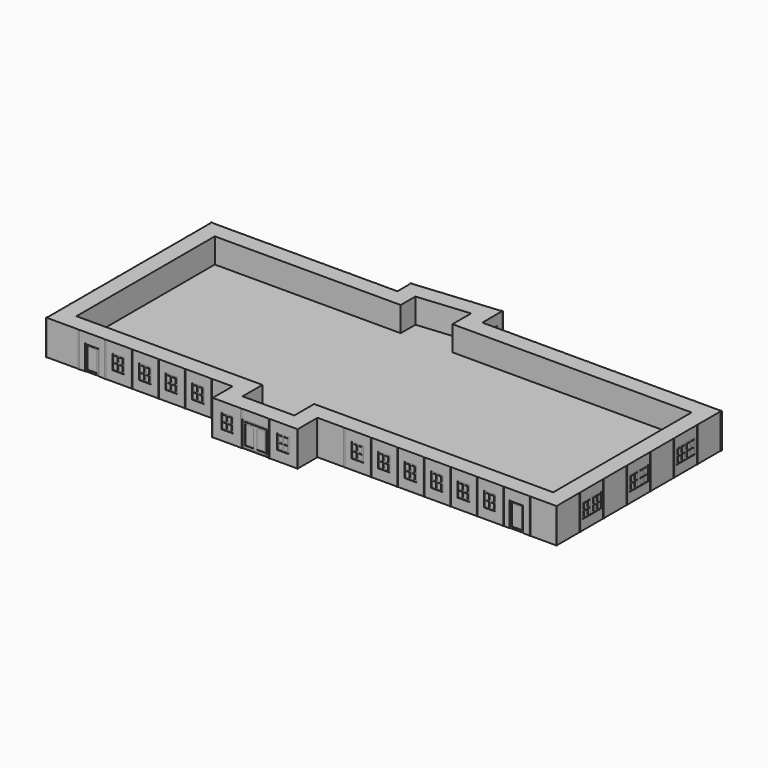
from build123d import *

# Parameters (mm, degrees)
F1_DEPTH  = 42
F3_DEPTH  = 30
F4_W      = 1.6
F4_H      = 42
F4_W_2    = 0.8
F6_W      = 1.6
F6_H      = 42
F8_W      = 1.6
F8_H      = 42
F8_W_2    = 0.8
F16_DEPTH = 0.4
F5_W      = 0.8
F5_H      = 42
F5_W_2    = 1.6
F10_W     = 1.6
F10_H     = 42
F12_W     = 0.8
F12_H     = 42
F12_W_2   = 1.6
F17_DEPTH = 0.4
F7_W      = 0.8
F7_H      = 42
F7_W_2    = 1.6
F9_W      = 1.6
F9_H      = 42
F14_W     = 0.8
F14_H     = 42
F14_W_2   = 1.6
F18_DEPTH = 0.4
F11_W     = 1.6
F11_H     = 42
F11_W_2   = 0.8
F13_W     = 1.6
F13_H     = 42
F15_W     = 1.6
F15_H     = 42
F15_W_2   = 0.8
F19_DEPTH = 0.4
F20_W     = 14.1428571429
F20_H     = 18
F20_W_2   = 4.1785714286
F20_H_2   = 6.1071428571
F21_W     = 14.1428571429
F21_H     = 18
F21_W_2   = 4.1785714286
F21_H_2   = 6.1071428571
F22_W     = 14.1428571429
F22_H     = 18
F22_W_2   = 4.1785714286
F22_H_2   = 6.1071428571
F23_DEPTH = 0.5
F24_W     = 17
F24_H     = 30
F24_W_2   = 15
F24_H_2   = 28
F24_W_3   = 12
F24_H_3   = 25
F25_DEPTH = 0.5
F26_W     = 17
F26_H     = 30
F26_W_2   = 15
F26_H_2   = 28
F26_W_3   = 12
F26_H_3   = 25
F27_DEPTH = 0.5
F28_W     = 31.4
F28_H     = 31
F28_W_2   = 27.4
F28_H_2   = 27
F28_W_3   = 10
F28_H_3   = 23
F29_DEPTH = 0.5
F32_W     = 14.1428571429
F32_H     = 18
F32_W_2   = 4.1785714286
F32_H_2   = 6.1071428571
F31_W     = 14.1428571429
F31_H     = 18
F31_W_2   = 4.1785714286
F31_H_2   = 6.1071428571
F30_W     = 14.1428571429
F30_H     = 18
F30_W_2   = 4.1785714286
F30_H_2   = 6.1071428571
F33_DEPTH = 0.5
F34_W     = 17
F34_H     = 30
F34_W_2   = 15
F34_H_2   = 28
F34_W_3   = 12
F34_H_3   = 25
F35_DEPTH = 0.5
F36_W     = 14.1428571429
F36_H     = 18
F36_W_2   = 4.1785714286
F36_H_2   = 6.1071428571
F37_W     = 30.4
F37_H     = 31
F37_W_2   = 26.4
F37_H_2   = 27
F37_W_3   = 10
F37_H_3   = 23
F38_DEPTH = 0.5
F39_W     = 4.1785714286
F39_H     = 6.1071428571
F39_W_2   = 14.1428571429
F39_H_2   = 18
F40_DEPTH = 0.5
F41_W     = 14.1428571429
F41_H     = 18
F41_W_2   = 4.1785714286
F41_H_2   = 6.1071428571
F42_DEPTH = 0.5
F43_W     = 14.1428571429
F43_H     = 18
F43_W_2   = 4.1785714286
F43_H_2   = 6.1071428571
F44_DEPTH = 0.5


# Not quite as in the source:
# - a feature names something its author has since deleted; it is built from what else it names


with BuildPart() as f1:
    # F0 (on Top) → F1 (new body)
    with BuildSketch(Plane.XY):
        Polygon((-327.3, 108.1424002851), (-327.3, -140.8575997149), (-102.6, -140.8575997149), (-102.6, -170.8575997149), (0, -170.8575997149), (0, -140.8575997149), (288.9, -140.8575997149), (288.9, 108.1424002851), (0, 108.1424002851), (0, 138.1424002851), (-102.6, 128.6424002851), (-102.6, 108.1424002851), align=None)
    extrude(amount=F1_DEPTH)

    # F2 (on face) → F3 (cut)
    with BuildSketch(Plane.XY.offset(42)):
        Polygon((-20, 88.1424002851), (-20, 116.2049975252), (-82.6, 110.4087012289), (-82.6, 88.1424002851), (-307.3, 88.1424002851), (-307.3, -120.8575997149), (-82.6, -120.8575997149), (-82.6, -150.8575997149), (-20, -150.8575997149), (-20, -120.8575997149), (268.9, -120.8575997149), (268.9, 88.1424002851), align=None)
    extrude(amount=-F3_DEPTH, mode=Mode.SUBTRACT)

    # F4 (on face) + F6 (on face) + F8 (on face) → F16 (join)
    with BuildSketch(Plane.XZ.offset(140.8575997149)):
        with Locations((-288.375, 21)):
            Rectangle(F4_W, F4_H)
        with Locations((-256.375, 21)):
            Rectangle(F4_W, F4_H)
        with Locations((-224.375, 21)):
            Rectangle(F4_W, F4_H)
        with Locations((-192.375, 21)):
            Rectangle(F4_W, F4_H)
        with Locations((-160.375, 21)):
            Rectangle(F4_W, F4_H)
        with Locations((-128.375, 21)):
            Rectangle(F4_W, F4_H)
        with Locations((-103, 21)):
            Rectangle(F4_W_2, F4_H)
        with Locations((-326.9, 21)):
            Rectangle(F4_W, F4_H)
    with BuildSketch(Plane.XZ.offset(170.8575997149)):
        with Locations((-102.2, 21)):
            Rectangle(F6_W, F6_H)
        with Locations((-0.4, 21)):
            Rectangle(F6_W, F6_H)
        with Locations((-34.8, 21)):
            Rectangle(F6_W, F6_H)
        with Locations((-67.8, 21)):
            Rectangle(F6_W, F6_H)
    with BuildSketch(Plane.XZ.offset(140.8575997149)):
        with Locations((288.5, 21)):
            Rectangle(F8_W, F8_H)
        with Locations((256.5, 21)):
            Rectangle(F8_W, F8_H)
        with Locations((224.5, 21)):
            Rectangle(F8_W, F8_H)
        with Locations((192.5, 21)):
            Rectangle(F8_W, F8_H)
        with Locations((160.5, 21)):
            Rectangle(F8_W, F8_H)
        with Locations((128.5, 21)):
            Rectangle(F8_W, F8_H)
        with Locations((96.5, 21)):
            Rectangle(F8_W, F8_H)
        with Locations((64.5, 21)):
            Rectangle(F8_W, F8_H)
        with Locations((32.5, 21)):
            Rectangle(F8_W, F8_H)
        with Locations((0.4, 21)):
            Rectangle(F8_W_2, F8_H)
    extrude(amount=F16_DEPTH)

    # F5 (on face) + F10 (on face) + F12 (on face) → F17 (join)
    with BuildSketch(Plane(origin=(-102.6, 0, 0), x_dir=(0, -1, 0), z_dir=(-1, 0, 0))):
        with Locations((141.2575997149, 21)):
            Rectangle(F5_W, F5_H)
        with Locations((170.4575997149, 21)):
            Rectangle(F5_W_2, F5_H)
    with BuildSketch(Plane(origin=(-327.3, 0, 0), x_dir=(0, -1, 0), z_dir=(-1, 0, 0))):
        with Locations((-108.0424002851, 21)):
            Rectangle(F10_W, F10_H)
        with Locations((-72.5424002851, 21)):
            Rectangle(F10_W, F10_H)
        with Locations((-37.0424002851, 21)):
            Rectangle(F10_W, F10_H)
        with Locations((-1.5424002851, 21)):
            Rectangle(F10_W, F10_H)
        with Locations((33.9575997149, 21)):
            Rectangle(F10_W, F10_H)
        with Locations((69.4575997149, 21)):
            Rectangle(F10_W, F10_H)
        with Locations((104.9575997149, 21)):
            Rectangle(F10_W, F10_H)
        with Locations((140.4575997149, 21)):
            Rectangle(F10_W, F10_H)
    with BuildSketch(Plane(origin=(-102.6, 0, 0), x_dir=(0, -1, 0), z_dir=(-1, 0, 0))):
        with Locations((-108.5424002851, 21)):
            Rectangle(F12_W, F12_H)
        with Locations((-128.2424002851, 21)):
            Rectangle(F12_W_2, F12_H)
    extrude(amount=F17_DEPTH)

    # F7 (on face) + F9 (on face) + F14 (on face) → F18 (join)
    with BuildSketch(Plane.YZ):
        with Locations((-141.2575997149, 21)):
            Rectangle(F7_W, F7_H)
        with Locations((-170.4575997149, 21)):
            Rectangle(F7_W_2, F7_H)
    with BuildSketch(Plane.YZ.offset(288.9)):
        with Locations((-140.4575997149, 21)):
            Rectangle(F9_W, F9_H)
        with Locations((-105.0004568577, 21)):
            Rectangle(F9_W, F9_H)
        with Locations((-69.5433140006, 21)):
            Rectangle(F9_W, F9_H)
        with Locations((-34.0861711434, 21)):
            Rectangle(F9_W, F9_H)
        with Locations((1.3709717137, 21)):
            Rectangle(F9_W, F9_H)
        with Locations((36.8281145709, 21)):
            Rectangle(F9_W, F9_H)
        with Locations((72.285257428, 21)):
            Rectangle(F9_W, F9_H)
        with Locations((107.7424002851, 21)):
            Rectangle(F9_W, F9_H)
    with BuildSketch(Plane.YZ):
        with Locations((108.5424002851, 21)):
            Rectangle(F14_W, F14_H)
        with Locations((137.7792795694, 21)):
            Rectangle(F14_W_2, F14_H)
    extrude(amount=F18_DEPTH)

    # F11 (on face) + F13 (on face) + F15 (on face) → F19 (join)
    with BuildSketch(Plane(origin=(0, 108.1424002851, 0), x_dir=(-1, 0, 0), z_dir=(0, 1, 0))):
        with Locations((288.375, 21)):
            Rectangle(F11_W, F11_H)
        with Locations((256.375, 21)):
            Rectangle(F11_W, F11_H)
        with Locations((224.375, 21)):
            Rectangle(F11_W, F11_H)
        with Locations((192.375, 21)):
            Rectangle(F11_W, F11_H)
        with Locations((160.375, 21)):
            Rectangle(F11_W, F11_H)
        with Locations((128.375, 21)):
            Rectangle(F11_W, F11_H)
        with Locations((103, 21)):
            Rectangle(F11_W_2, F11_H)
        with Locations((326.9, 21)):
            Rectangle(F11_W, F11_H)
    with BuildSketch(Plane(origin=(-12.6822332802, 136.9681194259, 0), x_dir=(-0.9957406741, -0.0921982106, 0), z_dir=(-0.0921982106, 0.9957406741, 0))):
        with Locations((-12.3364821089, 21)):
            Rectangle(F13_W, F13_H)
        with Locations((89.8655147654, 21)):
            Rectangle(F13_W, F13_H)
        with Locations((22.2829559704, 21)):
            Rectangle(F13_W, F13_H)
        with Locations((55.2829559704, 21)):
            Rectangle(F13_W, F13_H)
    with BuildSketch(Plane(origin=(0, 108.1424002851, 0), x_dir=(-1, 0, 0), z_dir=(0, 1, 0))):
        with Locations((-288.5, 21)):
            Rectangle(F15_W, F15_H)
        with Locations((-256.5, 21)):
            Rectangle(F15_W, F15_H)
        with Locations((-224.5, 21)):
            Rectangle(F15_W, F15_H)
        with Locations((-192.5, 21)):
            Rectangle(F15_W, F15_H)
        with Locations((-160.5, 21)):
            Rectangle(F15_W, F15_H)
        with Locations((-128.5, 21)):
            Rectangle(F15_W, F15_H)
        with Locations((-96.5, 21)):
            Rectangle(F15_W, F15_H)
        with Locations((-64.5, 21)):
            Rectangle(F15_W, F15_H)
        with Locations((-32.5, 21)):
            Rectangle(F15_W, F15_H)
        with Locations((-0.4, 21)):
            Rectangle(F15_W_2, F15_H)
    extrude(amount=F19_DEPTH, dir=(0, 1, 0))

    # F20 (on face) + F21 (on face) + F22 (on face) → F23 (cut)
    with BuildSketch(Plane.XZ.offset(170.8575997149)):
        with Locations((-85.0000714286, 21)):
            Rectangle(F20_W, F20_H)
        with Locations((-88.0536428571, 16.9821428571)):
            Rectangle(F20_W_2, F20_H_2, mode=Mode.SUBTRACT)
        with Locations((-81.9465, 16.9821428571)):
            Rectangle(F20_W_2, F20_H_2, mode=Mode.SUBTRACT)
        with Locations((-88.0536428571, 25.0178571429)):
            Rectangle(F20_W_2, F20_H_2, mode=Mode.SUBTRACT)
        with Locations((-81.9465, 25.0178571429)):
            Rectangle(F20_W_2, F20_H_2, mode=Mode.SUBTRACT)
    with BuildSketch(Plane.XZ.offset(170.8575997149)):
        with Locations((-17.6000714286, 21)):
            Rectangle(F21_W, F21_H)
        with Locations((-20.6536428571, 16.9821428571)):
            Rectangle(F21_W_2, F21_H_2, mode=Mode.SUBTRACT)
        with Locations((-14.5465, 16.9821428571)):
            Rectangle(F21_W_2, F21_H_2, mode=Mode.SUBTRACT)
        with Locations((-20.6536428571, 25.0178571429)):
            Rectangle(F21_W_2, F21_H_2, mode=Mode.SUBTRACT)
        with Locations((-14.5465, 25.0178571429)):
            Rectangle(F21_W_2, F21_H_2, mode=Mode.SUBTRACT)
    with BuildSketch(Plane.XZ.offset(140.8575997149)):
        with Locations((-208.5035714286, 21)):
            Rectangle(F22_W, F22_H)
        with Locations((-211.5571428571, 16.9821428571)):
            Rectangle(F22_W_2, F22_H_2, mode=Mode.SUBTRACT)
        with Locations((-205.45, 16.9821428571)):
            Rectangle(F22_W_2, F22_H_2, mode=Mode.SUBTRACT)
        with Locations((-211.5571428571, 25.0178571429)):
            Rectangle(F22_W_2, F22_H_2, mode=Mode.SUBTRACT)
        with Locations((-205.45, 25.0178571429)):
            Rectangle(F22_W_2, F22_H_2, mode=Mode.SUBTRACT)
    extrude(amount=-F23_DEPTH, mode=Mode.SUBTRACT)

    # F24 (on face) → F25 (cut)
    with BuildSketch(Plane.XZ.offset(140.8575997149)):
        with Locations((-272.375, 15)):
            Rectangle(F24_W, F24_H)
        with Locations((-272.375, 15)):
            Rectangle(F24_W_2, F24_H_2, mode=Mode.SUBTRACT)
        with Locations((-272.375, 15)):
            Rectangle(F24_W_3, F24_H_3)
    extrude(amount=-F25_DEPTH, mode=Mode.SUBTRACT)

    # F26 (on face) → F27 (cut)
    with BuildSketch(Plane.XZ.offset(140.8575997149)):
        with Locations((240.5, 15)):
            Rectangle(F26_W, F26_H)
        with Locations((240.5, 15)):
            Rectangle(F26_W_2, F26_H_2, mode=Mode.SUBTRACT)
        with Locations((240.5, 15)):
            Rectangle(F26_W_3, F26_H_3)
    extrude(amount=-F27_DEPTH, mode=Mode.SUBTRACT)

    # F28 (on face) → F29 (cut)
    with BuildSketch(Plane.XZ.offset(170.8575997149)):
        with Locations((-51.3, 15.5)):
            Rectangle(F28_W, F28_H)
        with Locations((-51.3, 15.5)):
            Rectangle(F28_W_2, F28_H_2, mode=Mode.SUBTRACT)
        with Locations((-58.3882954717, 15.5)):
            Rectangle(F28_W_3, F28_H_3)
        with Locations((-44.3882938325, 15.5)):
            Rectangle(F28_W_3, F28_H_3)
    extrude(amount=-F29_DEPTH, mode=Mode.SUBTRACT)

    # F32 (on face) + F31 (on face) + F30 (on face) → F33 (cut)
    with BuildSketch(Plane.YZ.offset(288.9)):
        with Locations((47.4850431423, 21)):
            Rectangle(F32_W, F32_H)
        with Locations((44.4314717137, 16.9821428571)):
            Rectangle(F32_W_2, F32_H_2, mode=Mode.SUBTRACT)
        with Locations((50.5386145709, 16.9821428571)):
            Rectangle(F32_W_2, F32_H_2, mode=Mode.SUBTRACT)
        with Locations((44.4314717137, 25.0178571429)):
            Rectangle(F32_W_2, F32_H_2, mode=Mode.SUBTRACT)
        with Locations((50.5386145709, 25.0178571429)):
            Rectangle(F32_W_2, F32_H_2, mode=Mode.SUBTRACT)
        with Locations((61.6279002851, 21)):
            Rectangle(F32_W, F32_H)
        with Locations((58.5743288566, 16.9821428571)):
            Rectangle(F32_W_2, F32_H_2, mode=Mode.SUBTRACT)
        with Locations((64.6814717137, 16.9821428571)):
            Rectangle(F32_W_2, F32_H_2, mode=Mode.SUBTRACT)
        with Locations((58.5743288566, 25.0178571429)):
            Rectangle(F32_W_2, F32_H_2, mode=Mode.SUBTRACT)
        with Locations((64.6814717137, 25.0178571429)):
            Rectangle(F32_W_2, F32_H_2, mode=Mode.SUBTRACT)
    with BuildSketch(Plane.YZ.offset(288.9)):
        with Locations((-23.429242572, 21)):
            Rectangle(F31_W, F31_H)
        with Locations((-26.4828140006, 16.9821428571)):
            Rectangle(F31_W_2, F31_H_2, mode=Mode.SUBTRACT)
        with Locations((-20.3756711434, 16.9821428571)):
            Rectangle(F31_W_2, F31_H_2, mode=Mode.SUBTRACT)
        with Locations((-26.4828140006, 25.0178571429)):
            Rectangle(F31_W_2, F31_H_2, mode=Mode.SUBTRACT)
        with Locations((-20.3756711434, 25.0178571429)):
            Rectangle(F31_W_2, F31_H_2, mode=Mode.SUBTRACT)
        with Locations((-9.2863854291, 21)):
            Rectangle(F31_W, F31_H)
        with Locations((-12.3399568577, 16.9821428571)):
            Rectangle(F31_W_2, F31_H_2, mode=Mode.SUBTRACT)
        with Locations((-6.2328140006, 16.9821428571)):
            Rectangle(F31_W_2, F31_H_2, mode=Mode.SUBTRACT)
        with Locations((-12.3399568577, 25.0178571429)):
            Rectangle(F31_W_2, F31_H_2, mode=Mode.SUBTRACT)
        with Locations((-6.2328140006, 25.0178571429)):
            Rectangle(F31_W_2, F31_H_2, mode=Mode.SUBTRACT)
    with BuildSketch(Plane.YZ.offset(288.9)):
        with Locations((-94.3435282863, 21)):
            Rectangle(F30_W, F30_H)
        with Locations((-97.3970997149, 16.9821428571)):
            Rectangle(F30_W_2, F30_H_2, mode=Mode.SUBTRACT)
        with Locations((-91.2899568577, 16.9821428571)):
            Rectangle(F30_W_2, F30_H_2, mode=Mode.SUBTRACT)
        with Locations((-97.3970997149, 25.0178571429)):
            Rectangle(F30_W_2, F30_H_2, mode=Mode.SUBTRACT)
        with Locations((-91.2899568577, 25.0178571429)):
            Rectangle(F30_W_2, F30_H_2, mode=Mode.SUBTRACT)
        with Locations((-80.2006711434, 21)):
            Rectangle(F30_W, F30_H)
        with Locations((-83.254242572, 16.9821428571)):
            Rectangle(F30_W_2, F30_H_2, mode=Mode.SUBTRACT)
        with Locations((-77.1470997149, 16.9821428571)):
            Rectangle(F30_W_2, F30_H_2, mode=Mode.SUBTRACT)
        with Locations((-83.254242572, 25.0178571429)):
            Rectangle(F30_W_2, F30_H_2, mode=Mode.SUBTRACT)
        with Locations((-77.1470997149, 25.0178571429)):
            Rectangle(F30_W_2, F30_H_2, mode=Mode.SUBTRACT)
    extrude(amount=-F33_DEPTH, mode=Mode.SUBTRACT)

    # F34 (on face) → F35 (cut)
    with BuildSketch(Plane.YZ):
        with Locations((122.9608399273, 15)):
            Rectangle(F34_W, F34_H)
        with Locations((122.9608399273, 15)):
            Rectangle(F34_W_2, F34_H_2, mode=Mode.SUBTRACT)
        with Locations((122.9608399273, 15)):
            Rectangle(F34_W_3, F34_H_3)
    extrude(amount=-F35_DEPTH, mode=Mode.SUBTRACT)

    # F36 (on face) + F37 (on face) → F38 (cut)
    with BuildSketch(Plane(origin=(-12.6822332802, 136.9681194259, 0), x_dir=(-0.9957406741, -0.0921982106, 0), z_dir=(-0.0921982106, 0.9957406741, 0))):
        with Locations((38.0461481147, 21)):
            Rectangle(F36_W, F36_H)
        with Locations((34.9925766862, 16.9821428571)):
            Rectangle(F36_W_2, F36_H_2, mode=Mode.SUBTRACT)
        with Locations((41.0997195433, 16.9821428571)):
            Rectangle(F36_W_2, F36_H_2, mode=Mode.SUBTRACT)
        with Locations((34.9925766862, 25.0178571429)):
            Rectangle(F36_W_2, F36_H_2, mode=Mode.SUBTRACT)
        with Locations((41.0997195433, 25.0178571429)):
            Rectangle(F36_W_2, F36_H_2, mode=Mode.SUBTRACT)
        with Locations((5.0461481147, 21)):
            Rectangle(F36_W, F36_H)
        with Locations((1.9925766862, 16.9821428571)):
            Rectangle(F36_W_2, F36_H_2, mode=Mode.SUBTRACT)
        with Locations((8.0997195433, 16.9821428571)):
            Rectangle(F36_W_2, F36_H_2, mode=Mode.SUBTRACT)
        with Locations((1.9925766862, 25.0178571429)):
            Rectangle(F36_W_2, F36_H_2, mode=Mode.SUBTRACT)
        with Locations((8.0997195433, 25.0178571429)):
            Rectangle(F36_W_2, F36_H_2, mode=Mode.SUBTRACT)
        with Locations((72.4460052576, 21)):
            Rectangle(F36_W, F36_H)
        with Locations((69.392433829, 16.9821428571)):
            Rectangle(F36_W_2, F36_H_2, mode=Mode.SUBTRACT)
        with Locations((75.4995766862, 16.9821428571)):
            Rectangle(F36_W_2, F36_H_2, mode=Mode.SUBTRACT)
        with Locations((69.392433829, 25.0178571429)):
            Rectangle(F36_W_2, F36_H_2, mode=Mode.SUBTRACT)
        with Locations((75.4995766862, 25.0178571429)):
            Rectangle(F36_W_2, F36_H_2, mode=Mode.SUBTRACT)
    with BuildSketch(Plane(origin=(0, 108.1424002851, 0), x_dir=(-1, 0, 0), z_dir=(0, 1, 0))):
        with Locations((272.375, 15.5)):
            Rectangle(F37_W, F37_H)
        with Locations((272.375, 15.5)):
            Rectangle(F37_W_2, F37_H_2, mode=Mode.SUBTRACT)
        with Locations((265.7867045283, 15.5)):
            Rectangle(F37_W_3, F37_H_3)
        with Locations((279.7867061675, 15.5)):
            Rectangle(F37_W_3, F37_H_3)
    extrude(amount=-F38_DEPTH, dir=(-0.0921982106, 0.9957406741, 0), mode=Mode.SUBTRACT)

    # F39 (on face) → F40 (cut)
    with BuildSketch(Plane.XZ.offset(140.8575997149)):
        Polygon((-233.4321428571, 30), (-247.575, 30), (-247.575, 12), (-233.4321428571, 12), (-233.4321428571, 12.718715705), align=None)
        with Locations((-243.5571428571, 16.9821428571)):
            Rectangle(F39_W, F39_H, mode=Mode.SUBTRACT)
        with Locations((-237.45, 16.9821428571)):
            Rectangle(F39_W, F39_H, mode=Mode.SUBTRACT)
        with Locations((-243.5571428571, 25.0178571429)):
            Rectangle(F39_W, F39_H, mode=Mode.SUBTRACT)
        with Locations((-237.45, 25.0178571429)):
            Rectangle(F39_W, F39_H, mode=Mode.SUBTRACT)
        with Locations((-176.5035714286, 21)):
            Rectangle(F39_W_2, F39_H_2)
        with Locations((-179.5571428571, 16.9821428571)):
            Rectangle(F39_W, F39_H, mode=Mode.SUBTRACT)
        with Locations((-173.45, 16.9821428571)):
            Rectangle(F39_W, F39_H, mode=Mode.SUBTRACT)
        with Locations((-179.5571428571, 25.0178571429)):
            Rectangle(F39_W, F39_H, mode=Mode.SUBTRACT)
        with Locations((-173.45, 25.0178571429)):
            Rectangle(F39_W, F39_H, mode=Mode.SUBTRACT)
        Polygon((-137.4321428571, 30), (-151.575, 30), (-151.575, 12), (-137.4321428571, 12), (-137.4321428571, 18.3077804595), align=None)
        with Locations((-147.5571428571, 16.9821428571)):
            Rectangle(F39_W, F39_H, mode=Mode.SUBTRACT)
        with Locations((-141.45, 16.9821428571)):
            Rectangle(F39_W, F39_H, mode=Mode.SUBTRACT)
        with Locations((-147.5571428571, 25.0178571429)):
            Rectangle(F39_W, F39_H, mode=Mode.SUBTRACT)
        with Locations((-141.45, 25.0178571429)):
            Rectangle(F39_W, F39_H, mode=Mode.SUBTRACT)
    extrude(amount=-F40_DEPTH, mode=Mode.SUBTRACT)

    # F41 (on face) → F42 (cut)
    with BuildSketch(Plane.XZ.offset(140.8575997149)):
        with Locations((48.3714285714, 21)):
            Rectangle(F41_W, F41_H)
        with Locations((45.3178571429, 16.9821428571)):
            Rectangle(F41_W_2, F41_H_2, mode=Mode.SUBTRACT)
        with Locations((51.425, 16.9821428571)):
            Rectangle(F41_W_2, F41_H_2, mode=Mode.SUBTRACT)
        with Locations((45.3178571429, 25.0178571429)):
            Rectangle(F41_W_2, F41_H_2, mode=Mode.SUBTRACT)
        with Locations((51.425, 25.0178571429)):
            Rectangle(F41_W_2, F41_H_2, mode=Mode.SUBTRACT)
        with Locations((80.3714285714, 21)):
            Rectangle(F41_W, F41_H)
        with Locations((77.3178571429, 16.9821428571)):
            Rectangle(F41_W_2, F41_H_2, mode=Mode.SUBTRACT)
        with Locations((83.425, 16.9821428571)):
            Rectangle(F41_W_2, F41_H_2, mode=Mode.SUBTRACT)
        with Locations((77.3178571429, 25.0178571429)):
            Rectangle(F41_W_2, F41_H_2, mode=Mode.SUBTRACT)
        with Locations((83.425, 25.0178571429)):
            Rectangle(F41_W_2, F41_H_2, mode=Mode.SUBTRACT)
        with Locations((112.3714285714, 21)):
            Rectangle(F41_W, F41_H)
        with Locations((109.3178571429, 16.9821428571)):
            Rectangle(F41_W_2, F41_H_2, mode=Mode.SUBTRACT)
        with Locations((115.425, 16.9821428571)):
            Rectangle(F41_W_2, F41_H_2, mode=Mode.SUBTRACT)
        with Locations((109.3178571429, 25.0178571429)):
            Rectangle(F41_W_2, F41_H_2, mode=Mode.SUBTRACT)
        with Locations((115.425, 25.0178571429)):
            Rectangle(F41_W_2, F41_H_2, mode=Mode.SUBTRACT)
        with Locations((144.3714285714, 21)):
            Rectangle(F41_W, F41_H)
        with Locations((141.3178571429, 16.9821428571)):
            Rectangle(F41_W_2, F41_H_2, mode=Mode.SUBTRACT)
        with Locations((147.425, 16.9821428571)):
            Rectangle(F41_W_2, F41_H_2, mode=Mode.SUBTRACT)
        with Locations((141.3178571429, 25.0178571429)):
            Rectangle(F41_W_2, F41_H_2, mode=Mode.SUBTRACT)
        with Locations((147.425, 25.0178571429)):
            Rectangle(F41_W_2, F41_H_2, mode=Mode.SUBTRACT)
        with Locations((176.3714285714, 21)):
            Rectangle(F41_W, F41_H)
        with Locations((173.3178571429, 16.9821428571)):
            Rectangle(F41_W_2, F41_H_2, mode=Mode.SUBTRACT)
        with Locations((179.425, 16.9821428571)):
            Rectangle(F41_W_2, F41_H_2, mode=Mode.SUBTRACT)
        with Locations((173.3178571429, 25.0178571429)):
            Rectangle(F41_W_2, F41_H_2, mode=Mode.SUBTRACT)
        with Locations((179.425, 25.0178571429)):
            Rectangle(F41_W_2, F41_H_2, mode=Mode.SUBTRACT)
        Polygon((215.4428571429, 30), (201.3, 30), (201.3, 12), (215.4428571429, 12), (215.4428571429, 13.5066565126), align=None)
        with Locations((205.3178571429, 16.9821428571)):
            Rectangle(F41_W_2, F41_H_2, mode=Mode.SUBTRACT)
        with Locations((211.425, 16.9821428571)):
            Rectangle(F41_W_2, F41_H_2, mode=Mode.SUBTRACT)
        with Locations((205.3178571429, 25.0178571429)):
            Rectangle(F41_W_2, F41_H_2, mode=Mode.SUBTRACT)
        with Locations((211.425, 25.0178571429)):
            Rectangle(F41_W_2, F41_H_2, mode=Mode.SUBTRACT)
    extrude(amount=-F42_DEPTH, mode=Mode.SUBTRACT)

    # F43 (on face) → F44 (cut)
    with BuildSketch(Plane(origin=(0, 108.1424002851, 0), x_dir=(-1, 0, 0), z_dir=(0, 1, 0))):
        with Locations((-208.6285714286, 21)):
            Rectangle(F43_W, F43_H)
        with Locations((-211.6821428571, 16.9821428571)):
            Rectangle(F43_W_2, F43_H_2, mode=Mode.SUBTRACT)
        with Locations((-205.575, 16.9821428571)):
            Rectangle(F43_W_2, F43_H_2, mode=Mode.SUBTRACT)
        with Locations((-211.6821428571, 25.0178571429)):
            Rectangle(F43_W_2, F43_H_2, mode=Mode.SUBTRACT)
        with Locations((-205.575, 25.0178571429)):
            Rectangle(F43_W_2, F43_H_2, mode=Mode.SUBTRACT)
        with Locations((-176.6285714286, 21)):
            Rectangle(F43_W, F43_H)
        with Locations((-179.6821428571, 16.9821428571)):
            Rectangle(F43_W_2, F43_H_2, mode=Mode.SUBTRACT)
        with Locations((-173.575, 16.9821428571)):
            Rectangle(F43_W_2, F43_H_2, mode=Mode.SUBTRACT)
        with Locations((-179.6821428571, 25.0178571429)):
            Rectangle(F43_W_2, F43_H_2, mode=Mode.SUBTRACT)
        with Locations((-173.575, 25.0178571429)):
            Rectangle(F43_W_2, F43_H_2, mode=Mode.SUBTRACT)
        Polygon((-137.5571428571, 30), (-151.7, 30), (-151.7, 12), (-137.5571428571, 12), (-137.5571428571, 12.1485680193), align=None)
        with Locations((-147.6821428571, 16.9821428571)):
            Rectangle(F43_W_2, F43_H_2, mode=Mode.SUBTRACT)
        with Locations((-141.575, 16.9821428571)):
            Rectangle(F43_W_2, F43_H_2, mode=Mode.SUBTRACT)
        with Locations((-147.6821428571, 25.0178571429)):
            Rectangle(F43_W_2, F43_H_2, mode=Mode.SUBTRACT)
        with Locations((-141.575, 25.0178571429)):
            Rectangle(F43_W_2, F43_H_2, mode=Mode.SUBTRACT)
        Polygon((-105.5571428571, 30), (-119.7, 30), (-119.7, 12), (-105.5571428571, 12), (-105.5571428571, 13.2916826606), align=None)
        with Locations((-115.6821428571, 16.9821428571)):
            Rectangle(F43_W_2, F43_H_2, mode=Mode.SUBTRACT)
        with Locations((-109.575, 16.9821428571)):
            Rectangle(F43_W_2, F43_H_2, mode=Mode.SUBTRACT)
        with Locations((-115.6821428571, 25.0178571429)):
            Rectangle(F43_W_2, F43_H_2, mode=Mode.SUBTRACT)
        with Locations((-109.575, 25.0178571429)):
            Rectangle(F43_W_2, F43_H_2, mode=Mode.SUBTRACT)
        Polygon((-73.5571428571, 30), (-87.7, 30), (-87.7, 12), (-73.5571428571, 12), (-73.5571428571, 13.5203055888), align=None)
        with Locations((-83.6821428571, 16.9821428571)):
            Rectangle(F43_W_2, F43_H_2, mode=Mode.SUBTRACT)
        with Locations((-77.575, 16.9821428571)):
            Rectangle(F43_W_2, F43_H_2, mode=Mode.SUBTRACT)
        with Locations((-83.6821428571, 25.0178571429)):
            Rectangle(F43_W_2, F43_H_2, mode=Mode.SUBTRACT)
        with Locations((-77.575, 25.0178571429)):
            Rectangle(F43_W_2, F43_H_2, mode=Mode.SUBTRACT)
    extrude(amount=-F44_DEPTH, mode=Mode.SUBTRACT)


solid = f1.part
